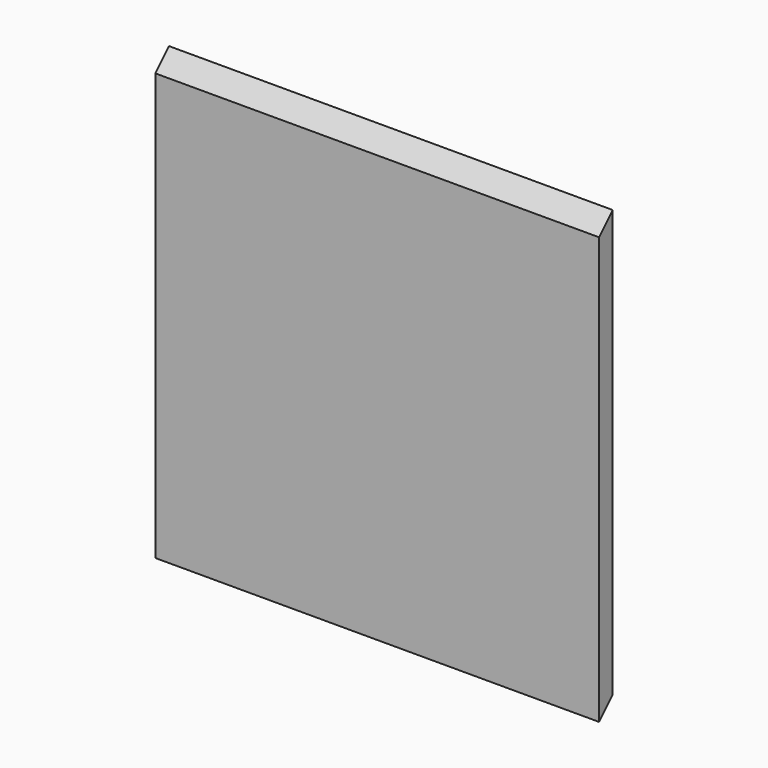
from build123d import *

# Parameters (mm, degrees)
F0_W     = 330.2
F0_H     = 12.7
F1_DEPTH = 330.2
F2_SIZE  = 12.69999


# Not quite as in the source:
# - a fillet or chamfer is up to 0.001 mm smaller than in the source, because OpenCascade refuses the exact size
# - a feature names something its author has since deleted; it is built from what else it names


with BuildPart() as f1:
    # F0 (on Top) → F1 (new body)
    with BuildSketch(Plane.XY):
        with Locations((132.5867457749, 25.1011773944)):
            Rectangle(F0_W, F0_H)
    extrude(amount=F1_DEPTH)

    # F2 (size 12.7 in the source; OpenCascade refuses exactly that, so slightly less here)
    f2_edges = [f1.edges().sort_by_distance(p)[0] for p in [
        (132.586746, 31.451177, 0),
        (132.586746, 18.751177, 330.2),
    ]]
    chamfer(f2_edges, length=F2_SIZE)


solid = f1.part
